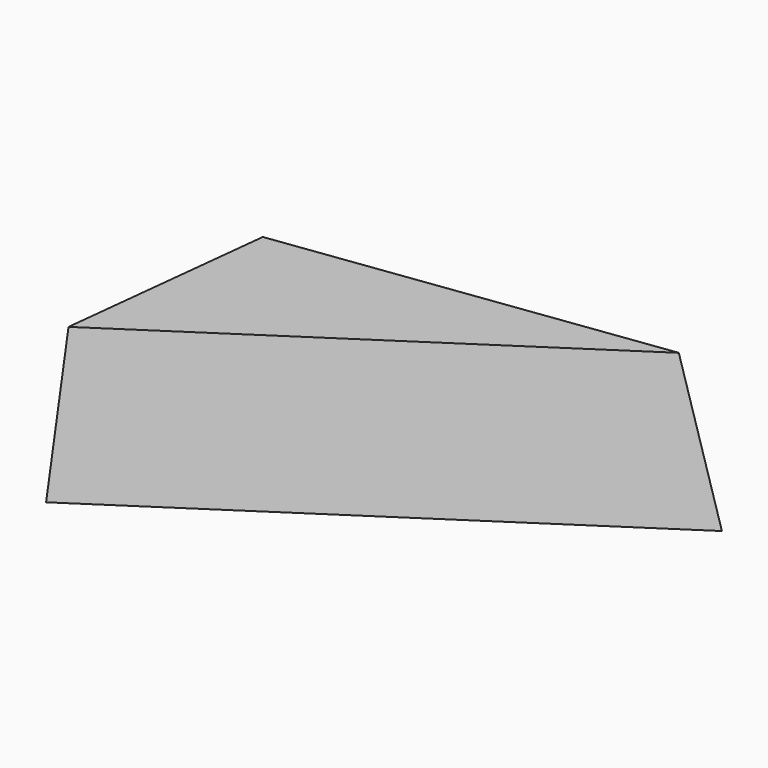
from build123d import *

# Parameters (mm, degrees)
F1_DEPTH = 25.4
F1_TAPER = 3


with BuildPart() as f1:
    # F0 (on Top) → F1 (new body)
    with BuildSketch(Plane.XY):
        Polygon((-44.0146140754, 10.6619251892), (-48.3887381852, -29.0696937591), (25.9713549167, 19.9569370598), align=None)
    extrude(amount=F1_DEPTH, taper=F1_TAPER)


solid = f1.part
